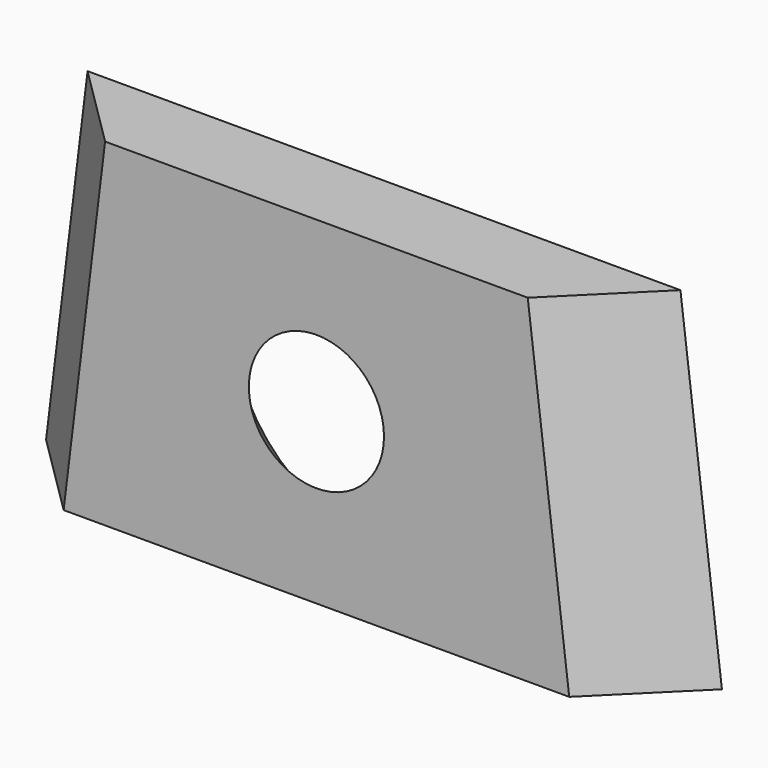
from build123d import *

# Parameters (mm, degrees)
F1_DEPTH = 3.175
F2_SIZE  = 3.17499
F3_R     = 2.54
F4_DEPTH = 25.4
F5_SIZE  = 3.17499


# Not quite as in the source:
# - a fillet or chamfer is up to 0.001 mm smaller than in the source, because OpenCascade refuses the exact size


with BuildPart() as f1:
    # F0 (on Front) → F1 (new body)
    with BuildSketch(Plane.XZ):
        Polygon((1.5593639235, 12.7), (0, 0), (25.4, 0), (23.8406360765, 12.7), align=None)
    extrude(amount=F1_DEPTH)

    # F2 (size 3.175 in the source; OpenCascade refuses exactly that, so slightly less here)
    f2_edges = [f1.edges().sort_by_distance(p)[0] for p in [
        (24.620318, -3.175, 6.35),
        (0.779682, -3.175, 6.35),
    ]]
    chamfer(f2_edges, length=F2_SIZE)

    # F3 (on face) → F4 (cut)
    with BuildSketch(Plane.XZ.offset(3.175)):
        with Locations((12.7, 6.35)):
            Circle(F3_R)
    extrude(amount=-F4_DEPTH, mode=Mode.SUBTRACT)

    # F5 (size 3.175 in the source; OpenCascade refuses exactly that, so slightly less here)
    f5_edges = [f1.edges().sort_by_distance(p)[0] for p in [
        (10.16, 0, 6.35),
    ]]
    chamfer(f5_edges, length=F5_SIZE)


solid = f1.part
